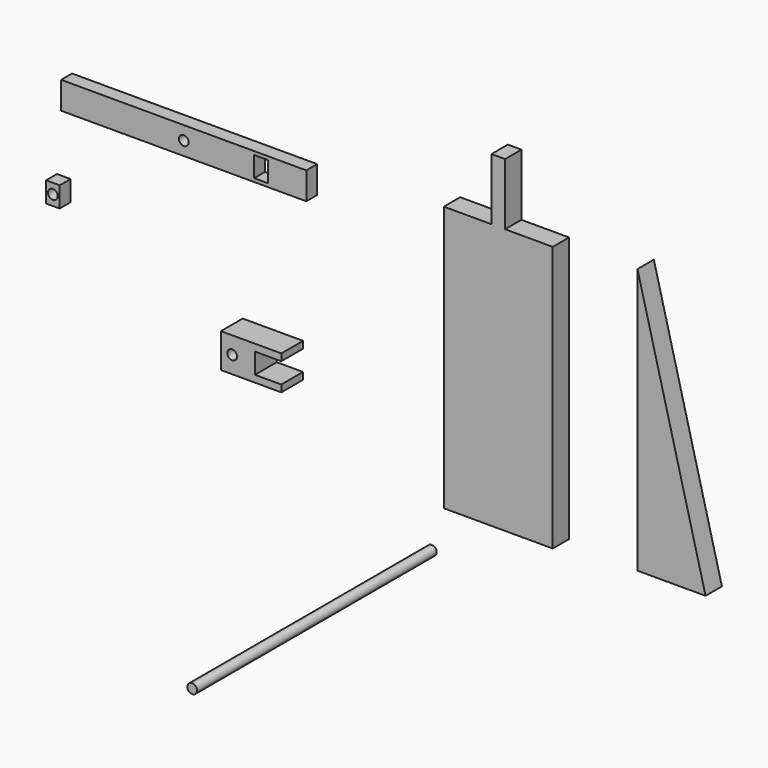
from build123d import *

# Parameters (mm, degrees)
F1_DEPTH = 20
F0_R     = 3.56
F2_DEPTH = 220
F0_W     = 180
F0_H     = 20
F0_W_2   = 10
F0_H_2   = 15
F3_DEPTH = 10
F4_DEPTH = 10
F5_DEPTH = 15
F6_DEPTH = 15


# Not quite as in the source:
# - a feature names something its author has since deleted; it is built from what else it names


with BuildPart() as f1:
    # F0 (on Front) → F1 (new body)
    with BuildSketch(Plane.XZ):
        with BuildLine():
            Line((-217.6441787565, 33.5391576588), (-217.6441787565, 38.6338087916))
            Line((-217.6441787565, 38.6338087916), (-236.9845063496, 38.6338087916))
            Line((-236.9845063496, 38.6338087916), (-236.9845063496, 53.6338087916))
            Line((-236.9845063496, 53.6338087916), (-217.6441787565, 53.6338087916))
            Line((-217.6441787565, 53.6338087916), (-217.6441787565, 58.7284599245))
            Line((-217.6441787565, 58.7284599245), (-253.6986111486, 58.7284599245))
            Line((-253.6986111486, 58.7284599245), (-253.6986111486, 49.6951619717))
            ThreePointArc((-253.6986111486, 49.6951619717), (-251.1803541648, 48.6520657755), (-250.1372579685, 46.1338087916))
            ThreePointArc((-250.1372579685, 46.1338087916), (-251.1803541648, 43.6155518078), (-253.6986111486, 42.5724556116))
            Line((-253.6986111486, 42.5724556116), (-253.6986111486, 33.5391576588))
            Line((-253.6986111486, 33.5391576588), (-217.6441787565, 33.5391576588))
        make_face()
        with BuildLine():
            Line((-261.9873631382, 33.5391576588), (-253.6986111486, 33.5391576588))
            Line((-253.6986111486, 33.5391576588), (-253.6986111486, 42.5724556116))
            ThreePointArc((-253.6986111486, 42.5724556116), (-257.2599643287, 46.1338087916), (-253.6986111486, 49.6951619717))
            Line((-253.6986111486, 49.6951619717), (-253.6986111486, 58.7284599245))
            Line((-253.6986111486, 58.7284599245), (-261.9873631382, 58.7284599245))
            Line((-261.9873631382, 58.7284599245), (-261.9873631382, 33.5391576588))
        make_face()
    extrude(amount=F1_DEPTH)


with BuildPart() as f2:
    # F0 (on Front) → F2 (new body)
    with BuildSketch(Plane.XZ):
        with Locations((-123.0808347464, -45.9383092821)):
            Circle(F0_R)
    extrude(amount=F2_DEPTH)


with BuildPart() as f3:
    # F0 (on Front) → F3 (new body)
    with BuildSketch(Plane.XZ):
        with Locations((-297.2545063496, 166.3678210974)):
            Rectangle(F0_W, F0_H)
        with Locations((-297.2545063496, 166.3678210974)):
            Circle(F0_R, mode=Mode.SUBTRACT)
        with Locations((-240.5445063496, 166.3678210974)):
            Rectangle(F0_W_2, F0_H_2, mode=Mode.SUBTRACT)
    extrude(amount=F3_DEPTH)


with BuildPart() as f4:
    # F0 (on Front) → F4 (new body)
    with BuildSketch(Plane.XZ):
        with Locations((-393.356616497, 100.299641192)):
            Rectangle(F0_W_2, F0_H_2)
        with Locations((-393.356616497, 100.299641192)):
            Circle(F0_R, mode=Mode.SUBTRACT)
    extrude(amount=F4_DEPTH)


with BuildPart() as f5:
    # F0 (on Front) → F5 (new body)
    with BuildSketch(Plane.XZ):
        Polygon((-102.3273542523, -5.9048458934), (-22.3273542523, -5.9048458934), (-22.3273542523, 189.0951541066), (-57.3273542523, 189.0951541066), (-62.3273542523, 189.0951541066), (-67.3273542523, 189.0951541066), (-102.3273542523, 189.0951541066), align=None)
        Polygon((-62.3273542523, 189.0951541066), (-57.3273542523, 189.0951541066), (-57.3273542523, 234.4632595778), (-67.3273542523, 234.4632595778), (-67.3273542523, 189.0951541066), align=None)
    extrude(amount=F5_DEPTH)


with BuildPart() as f5b:
    # F0 (on Front) → F5, piece 2 (new body)
    with BuildSketch(Plane.XZ):
        Polygon((89.8966632783, 0), (39.8966632783, 195), (39.8966632783, 0), align=None)
    extrude(amount=F5_DEPTH)


with BuildPart() as f6:
    # F0 (on Front) → F6 (new body)
    with BuildSketch(Plane.XZ):
        Polygon((89.8966632783, 0), (39.8966632783, 195), (39.8966632783, 0), align=None)
    extrude(amount=F6_DEPTH)


solid = Compound([f1.part, f2.part, f3.part, f4.part, f5.part, f5b.part, f6.part])
